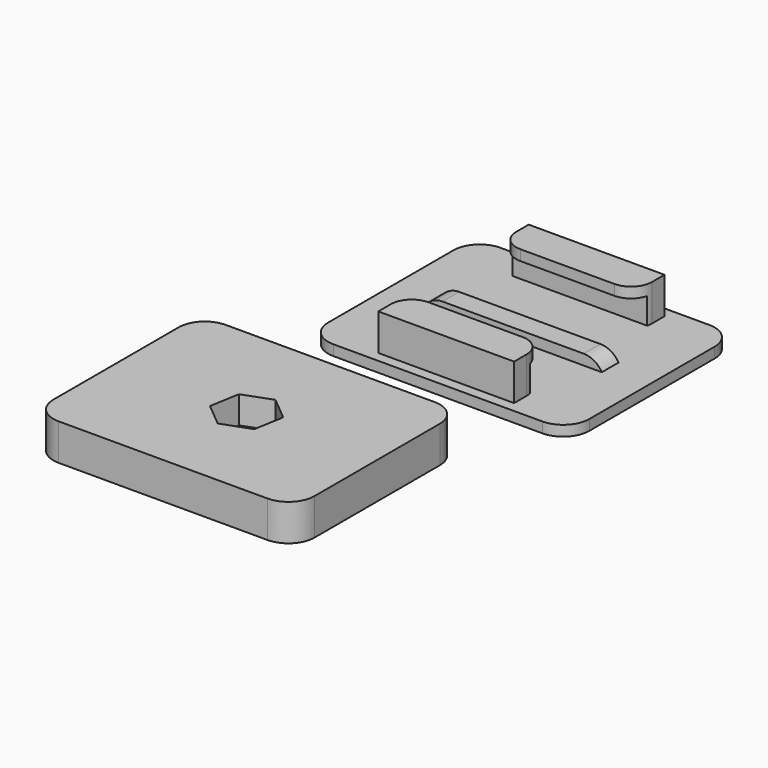
from build123d import *

# Parameters (mm, degrees)
F0_W           = 26
F0_H           = 4
F1_DEPTH       = 5
F2_W           = 26
F2_H           = 7
F3_DEPTH       = 2
F4_W           = 34
F4_H           = 4
F5_DEPTH       = 2
F6_W           = 50
F6_H           = 40
F7_DEPTH       = 2
F8_W           = 50
F8_H           = 40
F9_DEPTH       = 7
F11_R          = 3.5
F12_DEPTH      = 7.001
F13_DEPTH      = 5.25
F14_F1_R       = 4
F14_F2_R       = 4
F14_2_F1_R     = 4
F14_2_F2_R     = 4
F14_3_T1_DEPTH = 21.3205080757
F15_R          = 5
F16_R          = 5


# Not quite as in the source:
# - a fillet or chamfer that OpenCascade refuses, or shapes differently, is made with other operations: its cross-section is extruded or revolved along the edge and cut away or added


with BuildPart() as f1:
    # F0 (on Top) → F1 (new body)
    with BuildSketch(Plane.XY):
        with Locations((-13, 2)):
            Rectangle(F0_W, F0_H)
    extrude(amount=F1_DEPTH)

    # F2 (on face) → F3 (join)
    with BuildSketch(Plane.XY.offset(5)):
        with Locations((-13, 3.5)):
            Rectangle(F2_W, F2_H)
    extrude(amount=F3_DEPTH)

    # F14: fillet of radius 4 on 2 edges, made by hand

    # F14_f1
    f14_f1_edges = [f1.edges().sort_by_distance(p)[0] for p in [
        (0, 7, 6),
    ]]
    fillet(f14_f1_edges, radius=F14_F1_R)

    # F14_f2
    f14_f2_edges = [f1.edges().sort_by_distance(p)[0] for p in [
        (-26, 7, 6),
    ]]
    fillet(f14_f2_edges, radius=F14_F2_R)


with BuildPart() as f1b:
    # F0 (on Top) → F1, piece 2 (new body)
    with BuildSketch(Plane.XY):
        with Locations((-13, 34)):
            Rectangle(F0_W, F0_H)
    extrude(amount=F1_DEPTH)

    # F2 (on face) → F3, piece 2 (join)
    with BuildSketch(Plane.XY.offset(5)):
        with Locations((-13, 32.5)):
            Rectangle(F2_W, F2_H)
    extrude(amount=F3_DEPTH)

    # F14#2: fillet of radius 4 on 2 edges, made by hand

    # F14_2_f1
    f14_2_f1_edges = [f1b.edges().sort_by_distance(p)[0] for p in [
        (-26, 29, 6),
    ]]
    fillet(f14_2_f1_edges, radius=F14_2_F1_R)

    # F14_2_f2
    f14_2_f2_edges = [f1b.edges().sort_by_distance(p)[0] for p in [
        (0, 29, 6),
    ]]
    fillet(f14_2_f2_edges, radius=F14_2_F2_R)


with BuildPart() as f5:
    # F4 (on Top) → F5 (new body)
    with BuildSketch(Plane.XY):
        with Locations((-13, 18)):
            Rectangle(F4_W, F4_H)
    extrude(amount=F5_DEPTH)

    # F14#3: fillet of radius 4 on 2 edges, made by hand

    # F14_3_s2 → F14_3_t1 (cut)
    with BuildSketch(Plane.XZ.offset(-28.6602540378)):
        with BuildLine():
            ThreePointArc((4, 0), (2.5358983849, 1.4641016151), (0.5358983849, 2))
            Line((0.5358983849, 2), (4, 2))
            Line((4, 2), (4, 0))
        make_face()
        with BuildLine():
            ThreePointArc((-30, 0), (-28.5358983849, 1.4641016151), (-26.5358983849, 2))
            Line((-26.5358983849, 2), (-30, 2))
            Line((-30, 2), (-30, 0))
        make_face()
    extrude(amount=F14_3_T1_DEPTH, mode=Mode.SUBTRACT)


with BuildPart() as f7:
    # F6 (on Top) → F7 (new body)
    with BuildSketch(Plane.XY):
        with Locations((-13, 18)):
            Rectangle(F6_W, F6_H)
    extrude(amount=-F7_DEPTH)

    # F15
    f15_edges = [f7.edges().sort_by_distance(p)[0] for p in [
        (12, -2, -1),
        (12, 38, -1),
        (-38, -2, -1),
        (-38, 38, -1),
    ]]
    fillet(f15_edges, radius=F15_R)


with BuildPart() as f9:
    # F8 (on Top) → F9 (new body)
    with BuildSketch(Plane.XY):
        with Locations((-21.0967977971, -37.6512110233)):
            Rectangle(F8_W, F8_H)
    extrude(amount=F9_DEPTH)

    # F11 (on face) → F12 (cut, through all)
    with BuildSketch(Plane(origin=(0, 0, 0), x_dir=(1, 0, 0), z_dir=(0, 0, -1))):
        with Locations((-21.0967977971, 37.6512110233)):
            Circle(F11_R)
    extrude(amount=-F12_DEPTH, mode=Mode.SUBTRACT)

    # F10 (on face) → F13 (cut)
    with BuildSketch(Plane.XY.offset(7)):
        Polygon((-20.1108978699, -31.9625086522), (-25.5304086014, -33.9530454552), (-26.5163085287, -39.6417478263), (-22.0826977244, -43.3399133944), (-16.6631869928, -41.3493765914), (-15.6772870656, -35.6606742204), align=None)
    extrude(amount=-F13_DEPTH, mode=Mode.SUBTRACT)

    # F16
    f16_edges = [f9.edges().sort_by_distance(p)[0] for p in [
        (-46.096798, -17.651211, 3.5),
        (3.903202, -17.651211, 3.5),
        (-46.096798, -57.651211, 3.5),
        (3.903202, -57.651211, 3.5),
    ]]
    fillet(f16_edges, radius=F16_R)


solid = Compound([f1.part, f1b.part, f5.part, f7.part, f9.part])
